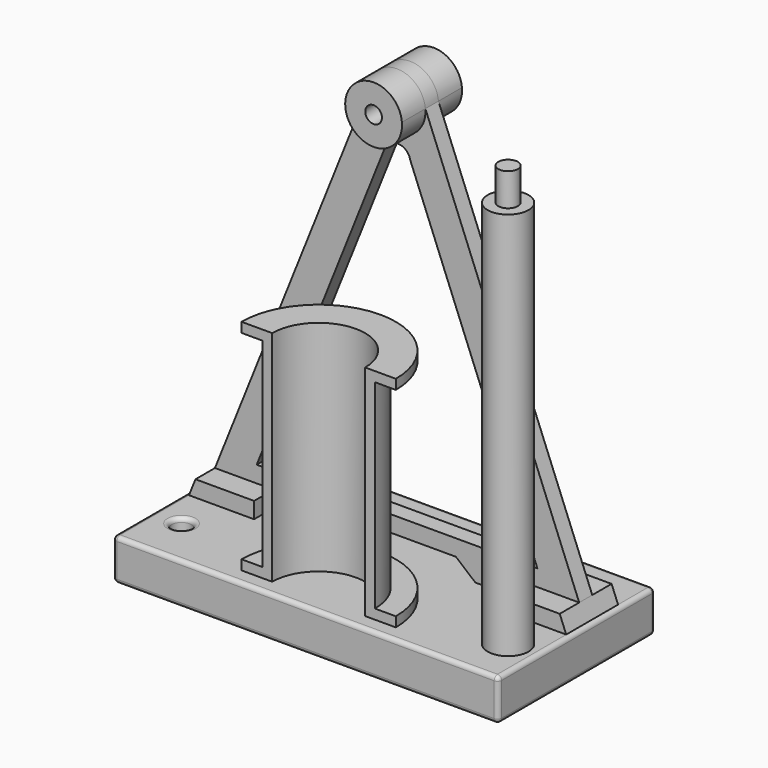
from build123d import *

# Parameters (mm, degrees)
F0_W      = 235.99902
F0_H      = 119.99976
F1_DEPTH  = 25.4
F2_R      = 5.99948
F3_DEPTH  = 40.386
F4_R      = 2.54
F6_R      = 5.10032
F7_DEPTH  = 9.99998
F8_DEPTH  = 14.80058
F9_DEPTH  = 24.89962
F10_DEPTH = 18.00098
F11_DEPTH = 27.94
F12_R     = 12.50061
F12_R_2   = 5.99948
F13_DEPTH = 238.00054
F14_DEPTH = 25.4
F15_R     = 5.99948
F16_DEPTH = 19.99996
F19_ANGLE = 180


# Not quite as in the source:
# - a feature names something its author has since deleted; it is built from what else it names


with BuildPart() as f1:
    # F0 (on Top) → F1 (new body)
    with BuildSketch(Plane.XY):
        Rectangle(F0_W, F0_H)
    extrude(amount=F1_DEPTH)

    # F2 (on face) → F3 (cut)
    with BuildSketch(Plane.XY.offset(25.4)):
        with Locations((-99.95789, -29.97962)):
            Circle(F2_R)
        with Locations((99.95789, -29.97962)):
            Circle(F2_R)
    extrude(amount=-F3_DEPTH, mode=Mode.SUBTRACT)

    # F4
    f4_edges = [f1.edges().sort_by_distance(p)[0] for p in [
        (0, -59.99988, 25.4),
        (117.99951, 0, 25.4),
        (0, 59.99988, 25.4),
        (-117.99951, -59.99988, 12.7),
        (117.99951, -59.99988, 12.7),
        (0, -59.99988, 0),
        (-117.99951, 0, 0),
        (117.99951, 0, 0),
        (0, 59.99988, 0),
        (-105.95737, -29.97962, 0),
        (93.95841, -29.97962, 0),
        (-117.99951, 59.99988, 12.7),
        (-117.99951, 0, 25.4),
        (117.99951, 59.99988, 12.7),
        (93.95841, -29.97962, 25.4),
        (105.95737, -29.97962, 12.7),
        (-105.95737, -29.97962, 25.4),
        (-93.95841, -29.97962, 12.7),
    ]]
    fillet(f4_edges, radius=F4_R)


with BuildPart() as f7:
    # F6 (on offset) → F7 (new body)
    with BuildSketch(Plane(origin=(0, 19.99996, 0), x_dir=(-1, 0, 0), z_dir=(0, 1, 0))):
        with BuildLine():
            ThreePointArc((17.3314493474, 270.8618911485), (0, 286.7161147099), (-17.3314493474, 270.8618911485))
            ThreePointArc((-17.3314493474, 270.8618911485), (-0.7737887103, 251.9327883875), (17.40027, 269.3158447099))
            ThreePointArc((17.40027, 269.3158447099), (17.3830563223, 270.0896334201), (17.3314493474, 270.8618911485))
        make_face()
        with Locations((0, 269.3158447099)):
            Circle(F6_R, mode=Mode.SUBTRACT)
        Polygon((-111.5014288749, 35.30092), (-115.45951, 25.4), (-75.60691, 25.4), (-75.60691, 35.30092), align=None)
        with BuildLine():
            Line((-75.60691, 35.30092), (-75.60691, 25.4))
            Line((-75.60691, 25.4), (-47.95647, 25.4))
            Line((-47.95647, 25.4), (-35.9959270127, 35.4360872093))
            Line((-35.9959270127, 35.4360872093), (0, 35.4360872093))
            Line((0, 35.4360872093), (35.9959270127, 35.4360872093))
            Line((35.9959270127, 35.4360872093), (47.95647, 25.4))
            Line((47.95647, 25.4), (75.60691, 25.4))
            Line((75.60691, 25.4), (75.60691, 35.30092))
            Line((75.60691, 35.30092), (111.5014288749, 35.30092))
            Line((111.5014288749, 35.30092), (17.3314493474, 270.8618911485))
            ThreePointArc((17.3314493474, 270.8618911485), (17.3830563223, 270.0896334201), (17.40027, 269.3158447099))
            ThreePointArc((17.40027, 269.3158447099), (-0.7737887103, 251.9327883875), (-17.3314493474, 270.8618911485))
            Line((-17.3314493474, 270.8618911485), (-111.5014288749, 35.30092))
            Line((-111.5014288749, 35.30092), (-75.60691, 35.30092))
        make_face()
        with BuildLine():
            Line((85.9252445798, 45.39996), (0, 45.39996))
            Line((0, 45.39996), (-85.9252445798, 45.39996))
            Line((-85.9252445798, 45.39996), (-8.0503976449, 240.1995624219))
            ThreePointArc((-8.0503976449, 240.1995624219), (-7.620364016, 241.7135981516), (-6.8881599273, 243.1068354916))
            ThreePointArc((-6.8881599273, 243.1068354916), (-3.8999689002, 245.7244062159), (0, 246.480187063))
            ThreePointArc((0, 246.480187063), (3.8999689002, 245.7244062159), (6.8881599273, 243.1068354916))
            ThreePointArc((6.8881599273, 243.1068354916), (7.620364016, 241.7135981516), (8.0503976449, 240.1995624219))
            Line((8.0503976449, 240.1995624219), (85.9252445798, 45.39996))
        make_face(mode=Mode.SUBTRACT)
        Polygon((115.45951, 25.4), (111.5014288749, 35.30092), (75.60691, 35.30092), (75.60691, 25.4), align=None)
    extrude(amount=-F7_DEPTH)

    # F6 (on offset) → F8 (join)
    with BuildSketch(Plane(origin=(0, 19.99996, 0), x_dir=(-1, 0, 0), z_dir=(0, 1, 0))):
        Polygon((-111.5014288749, 35.30092), (-115.45951, 25.4), (-75.60691, 25.4), (-75.60691, 35.30092), align=None)
        Polygon((115.45951, 25.4), (111.5014288749, 35.30092), (75.60691, 35.30092), (75.60691, 25.4), align=None)
    extrude(amount=F8_DEPTH)

    # F6 (on offset) → F9 (join)
    with BuildSketch(Plane(origin=(0, 19.99996, 0), x_dir=(-1, 0, 0), z_dir=(0, 1, 0))):
        Polygon((-111.5014288749, 35.30092), (-115.45951, 25.4), (-75.60691, 25.4), (-75.60691, 35.30092), align=None)
        Polygon((115.45951, 25.4), (111.5014288749, 35.30092), (75.60691, 35.30092), (75.60691, 25.4), align=None)
    extrude(amount=-F9_DEPTH)

    # F6 (on offset) → F10 (join)
    with BuildSketch(Plane(origin=(0, 19.99996, 0), x_dir=(-1, 0, 0), z_dir=(0, 1, 0))):
        with BuildLine():
            ThreePointArc((17.3314493474, 270.8618911485), (0, 286.7161147099), (-17.3314493474, 270.8618911485))
            ThreePointArc((-17.3314493474, 270.8618911485), (-0.7737887103, 251.9327883875), (17.40027, 269.3158447099))
            ThreePointArc((17.40027, 269.3158447099), (17.3830563223, 270.0896334201), (17.3314493474, 270.8618911485))
        make_face()
        with Locations((0, 269.3158447099)):
            Circle(F6_R, mode=Mode.SUBTRACT)
    extrude(amount=F10_DEPTH)

    # F6 (on offset) → F11 (join)
    with BuildSketch(Plane(origin=(0, 19.99996, 0), x_dir=(-1, 0, 0), z_dir=(0, 1, 0))):
        with BuildLine():
            ThreePointArc((17.3314493474, 270.8618911485), (0, 286.7161147099), (-17.3314493474, 270.8618911485))
            ThreePointArc((-17.3314493474, 270.8618911485), (-0.7737887103, 251.9327883875), (17.40027, 269.3158447099))
            ThreePointArc((17.40027, 269.3158447099), (17.3830563223, 270.0896334201), (17.3314493474, 270.8618911485))
        make_face()
        with Locations((0, 269.3158447099)):
            Circle(F6_R, mode=Mode.SUBTRACT)
    extrude(amount=-F11_DEPTH)


with BuildPart() as f13:
    # F12 (on face) → F13 (new body)
    with BuildSketch(Plane.XY.offset(25.4)):
        with Locations((99.95789, -29.97962)):
            Circle(F12_R)
        with Locations((99.95789, -29.97962)):
            Circle(F12_R_2, mode=Mode.SUBTRACT)
        with Locations((99.95789, -29.97962)):
            Circle(F12_R_2)
    extrude(amount=F13_DEPTH)

    # F12 (on face) → F14 (join, through all)
    with BuildSketch(Plane.XY.offset(25.4)):
        with Locations((99.95789, -29.97962)):
            Circle(F12_R_2)
    extrude(amount=-F14_DEPTH)

    # F15 (on face) → F16 (join)
    with BuildSketch(Plane.XY.offset(263.40054)):
        with Locations((99.95789, -29.97962)):
            Circle(F15_R)
    extrude(amount=F16_DEPTH)


with BuildPart() as f19:
    # F18 (on offset) → F19 (revolve)
    with BuildSketch(Plane.XZ.offset(49.9999)):
        Polygon((-47.2523905337, 31.39948), (-47.2523905337, 25.4), (-28.4513105337, 25.4), (-28.4513105337, 159.40024), (-47.2523905337, 159.40024), (-47.2523905337, 153.40076), (-34.4533305337, 153.40076), (-34.4533305337, 31.39948), align=None)
    revolve(axis=Axis((0, -49.9999, -8.691214025), (0, 0, -1)), revolution_arc=F19_ANGLE)


solid = Compound([f1.part, f7.part, f13.part, f19.part])
